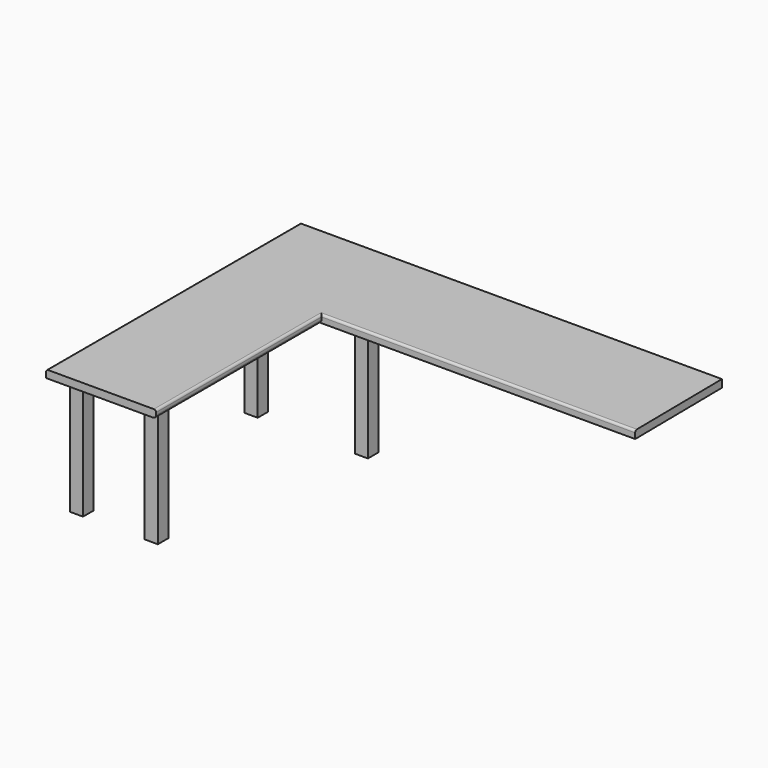
from build123d import *

# Parameters (mm, degrees)
F1_DEPTH = 44.45
F2_R     = 12.7
F3_R     = 17.78
F4_W     = 76.2
F4_H     = 76.2
F4_W_2   = 75.0966481864
F4_H_2   = 75.0966481864
F5_DEPTH = 685.8


# Not quite as in the source:
# - a feature names something its author has since deleted; it is built from what else it names


with BuildPart() as f1:
    # F0 (on Top) → F1 (new body)
    with BuildSketch(Plane.XY):
        Polygon((2406.7179050011, 1150.6131630864), (2399.3345719218, 1785.5702375352), (-39.0654280782, 1785.5702375352), (-39.0654280782, -43.2297624648), (595.9345719218, -43.2297624648), (595.9345719218, 1150.6131630864), align=None)
    extrude(amount=F1_DEPTH)

    # F2
    f2_edges = [f1.edges().sort_by_distance(p)[0] for p in [
        (595.934572, 553.6917, 44.45),
        (1501.326238, 1150.613163, 44.45),
        (-39.065428, 871.170238, 44.45),
    ]]
    fillet(f2_edges, radius=F2_R)

    # F3
    f3_edges = [f1.edges().sort_by_distance(p)[0] for p in [
        (595.934572, 553.6917, 0),
    ]]
    fillet(f3_edges, radius=F3_R)

    # F4 (on face) → F5 (join)
    with BuildSketch(Plane(origin=(0, 0, 0), x_dir=(1, 0, 0), z_dir=(0, 0, -1))):
        with Locations((75.2345719218, -71.0702375352)):
            Rectangle(F4_W, F4_H)
        with Locations((507.0345719218, -71.0702375352)):
            Rectangle(F4_W, F4_H)
        with Locations((723.7319641083, -1316.221913442)):
            Rectangle(F4_W_2, F4_H_2)
        with Locations((87.6286122948, -1316.221913442)):
            Rectangle(F4_W_2, F4_H_2)
    extrude(amount=F5_DEPTH)


solid = f1.part
